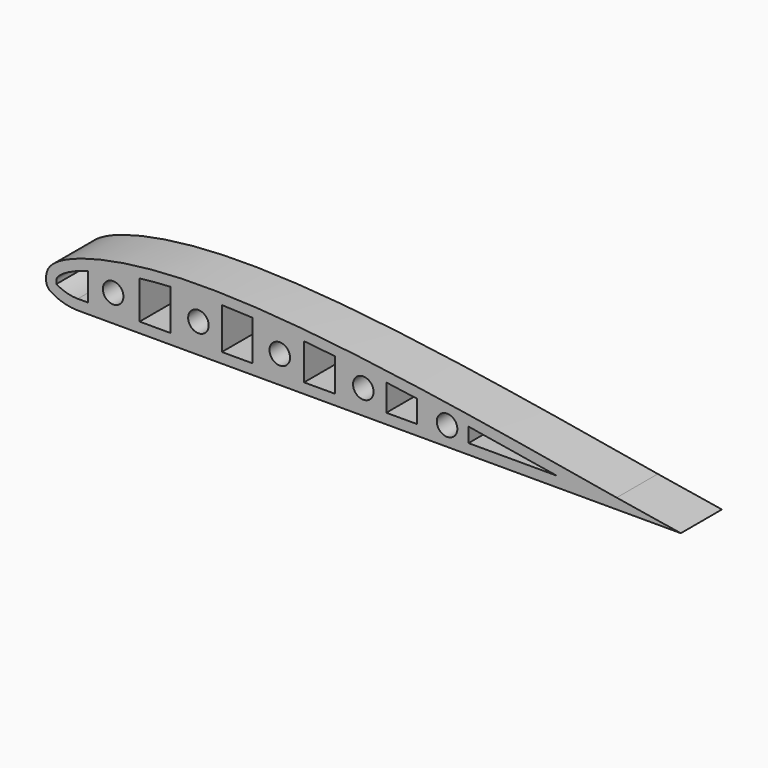
from build123d import *

# Parameters (mm, degrees)
F2_DEPTH    = 5
F3_R        = 5
F4_R        = 1
F5_T        = 1
F5_T3_DEPTH = 7
F6_DEPTH    = 25
F8_DEPTH    = 5
F9_DEPTH    = 5
F10_R       = 1
F11_DEPTH   = 25


# Not quite as in the source:
# - a shell that OpenCascade refuses in one call is made with other operations: the cavity is built on its own and cut out


with BuildPart() as f2:
    # F1 (on face) → F2 (new body)
    with BuildSketch(Plane.XZ):
        with BuildLine():
            Line((-26.5288872166, -15), (33.3456372568, -15))
            Line((33.3456372568, -15), (27.1073225886, -13.9837451279))
            add(Edge.make_bspline(
                [(-28.3359829336, -13.9837451279), (-28.4208510794, -13.3667707476), (-28.7214859578, -11.1812167846), (-13.7796289125, -6.9391380287), (10.881186874, -11.188066848), (27.1073225886, -13.9837451279)],
                knots=[0, 0, 0, 0, 0.1185783293, 0.420048799, 1, 1, 1, 1], degree=3))
            add(Edge.make_bspline(
                [(-26.5288872166, -15), (-26.86323879, -14.8644866499), (-27.537488468, -14.5823502704), (-28.0664619457, -14.1857962295), (-28.3359829336, -13.9837451279)],
                knots=[0.0540040051, 0.0540040051, 0.0540040051, 0.0540040051, 0.5179988224, 1, 1, 1, 1], degree=3))
        make_face()
    extrude(amount=F2_DEPTH)

    # F3
    f3_edges = [f2.edges().sort_by_distance(p)[0] for p in [
        (-26.528887, -2.5, -15),
    ]]
    fillet(f3_edges, radius=F3_R)

    # F4
    f4_edges = [f2.edges().sort_by_distance(p)[0] for p in [
        (-28.335983, -2.5, -13.983745),
    ]]
    fillet(f4_edges, radius=F4_R)

    # F5: shell of thickness 1, made by hand


with BuildPart() as f5_core1:
    # F5_t2: copy of F2
    add(f2.part)

    # the walls: a layer under each face that stays
    f5_faces = [f5_core1.faces().sort_by_distance(p)[0] for p in [
        (2.4583359072, 0, -10.9695690143),
        (-26.661850554, -2.5, -14.8149873071),
        (-28.2490657629, -2.5, -13.9382511648),
        (4.0156695071, -2.5, -15),
        (-10.6427774125, -2.5, -8.993895323),
        (30.2264799227, -2.5, -14.491872564),
    ]]
    thicken(f5_faces, amount=-F5_T, mode=Mode.SUBTRACT)

    # F5_s4 → F5_t3 (cut)
    with BuildSketch(Plane.XZ.offset(-1)):
        Polygon((27.1106283771, -13.9640204373), (26.9375295844, -14.9692248769), (26.9420297167, -14.9700002262), (26.9465367425, -14.9707344448), align=None)
    extrude(amount=F5_T3_DEPTH, mode=Mode.SUBTRACT)


with BuildPart() as f2_1:
    add(f2.part)

    # what is left inside the walls is the cavity
    f5_cavity = [f5_core1.part.solids().sort_by_distance(p)[0] for p in [
        (-12.827439, -3.666667, -9.966781),
    ]]
    add(f5_cavity, mode=Mode.SUBTRACT)

    # F6 (cut): a face of the model
    f6_faces = [f2_1.faces().sort_by_distance(p)[0] for p in [
        (-7.4171718542, -1, -12.3793689796),
    ]]
    extrude(f6_faces, amount=-F6_DEPTH, mode=Mode.SUBTRACT)

    # F7 (on Front) → F8 (join)
    with BuildSketch(Plane.XZ):
        Polygon((8.6958280578, -11.670999229), (7.6958280578, -11.6858640686), (7.6958280578, -14.3787935376), (8.6958280578, -14.2369903624), align=None)
        Polygon((-23.3041719422, -10.5932358738), (-24.3041719422, -10.7646555679), (-24.3041719422, -14.5308236647), (-23.3041719422, -14.6550234321), align=None)
        Polygon((-20.3041719422, -10.0012977139), (-20.3041719422, -14.4967306405), (-19.3041719422, -14.3338963389), (-19.3041719422, -9.9699208513), align=None)
        Polygon((-15.3041719422, -9.7202397883), (-16.3041719422, -9.8722195253), (-16.3041719422, -14.171061106), (-15.3041719422, -14.3121844158), align=None)
        Polygon((-11.3041719422, -9.5864236355), (-12.3041719422, -9.6656959504), (-12.3041719422, -14.2634715885), (-11.3041719422, -14.2337447032), align=None)
        Polygon((-7.3041719422, -9.6892677248), (-8.3041719422, -9.7621986642), (-8.3041719422, -14.2474444583), (-7.3041719422, -14.4419269636), align=None)
        Polygon((-3.3041719422, -10.0660771132), (-4.3041719422, -9.9566811696), (-4.3041719422, -14.1745144501), (-3.3041719422, -14.5391682163), align=None)
        Polygon((0.6958280578, -10.2848699316), (-0.3041719422, -10.3091802448), (-0.3041719422, -14.478392899), (0.6958280578, -14.49054759), align=None)
        Polygon((4.6958280578, -10.5765927583), (3.6958280578, -10.6495236978), (3.6958280578, -14.3811516464), (4.6958280578, -14.3933063373), align=None)
        Polygon((12.6958280578, -12.4591551721), (11.6958280578, -12.3501745984), (11.6958280578, -14.2489168793), (12.6958280578, -14.2280757427), align=None)
    extrude(amount=F8_DEPTH)

    # F7 (on Front) → F9 (join)
    with BuildSketch(Plane.XZ):
        Polygon((-12.3041719422, -9.6656959504), (-15.3041719422, -9.7202397883), (-15.3041719422, -14.3121844158), (-12.3041719422, -14.2634715885), align=None)
        Polygon((-4.3041719422, -9.9566811696), (-7.3041719422, -9.6892677248), (-7.3041719422, -14.4419269636), (-4.3041719422, -14.1745144501), align=None)
        Polygon((11.6958280578, -12.3501745984), (8.6958280578, -11.670999229), (8.6958280578, -14.2369903624), (11.6958280578, -14.2489168793), align=None)
        Polygon((-20.3041719422, -9.959064424), (-23.3041719422, -10.5932358738), (-23.3041719422, -14.6550234321), (-20.3041719422, -14.4967306405), (-20.3041719422, -10.0012977139), align=None)
        Polygon((3.6958280578, -10.6495236978), (0.6958280578, -10.2848699316), (0.6958280578, -14.49054759), (3.6958280578, -14.3811516464), align=None)
    extrude(amount=F9_DEPTH)

    # F10 (on face) → F11 (cut)
    with BuildSketch(Plane.XZ.offset(5)):
        with Locations((-21.8780643028, -12.3687916514)):
            Circle(F10_R)
        with Locations((-13.5824292234, -12.1407258353)):
            Circle(F10_R)
        with Locations((-5.6688322555, -12.330345645)):
            Circle(F10_R)
        with Locations((2.4586208165, -12.6149933785)):
            Circle(F10_R)
        with Locations((10.6068449969, -13.145046041)):
            Circle(F10_R)
    extrude(amount=-F11_DEPTH, mode=Mode.SUBTRACT)


solid = f2_1.part
